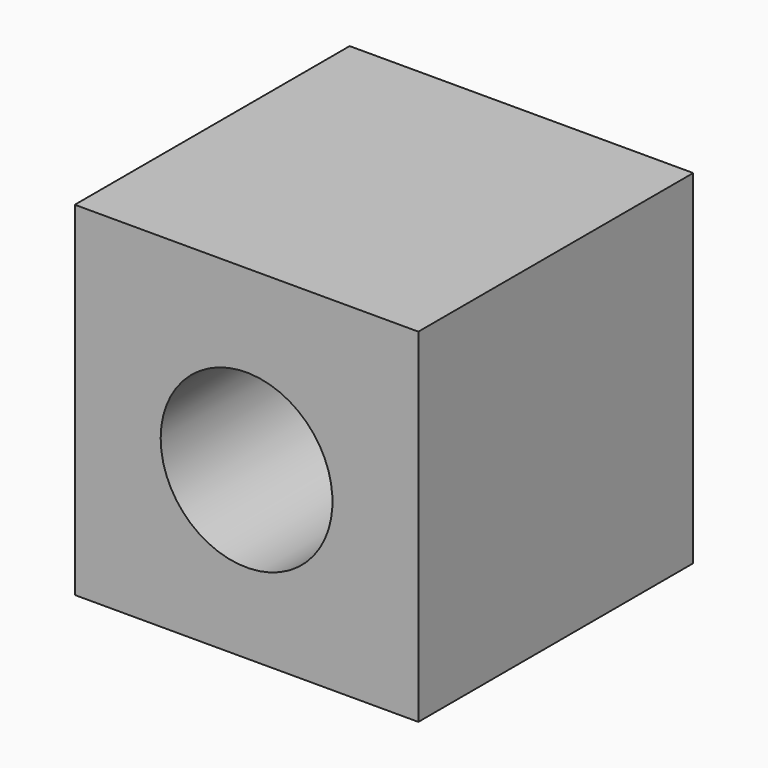
from build123d import *

# Parameters (mm, degrees)
F0_W     = 40
F0_H     = 40
F1_DEPTH = 40
F3_D     = 20


# Not quite as in the source:
# - a feature names something its author has since deleted; it is built from what else it names


with BuildPart() as f1:
    # F0 (on Front) → F1 (new body)
    with BuildSketch(Plane.XZ):
        with Locations((2.679047659, 0.6785862893)):
            Rectangle(F0_W, F0_H)
    extrude(amount=F1_DEPTH)

    # F3 (through all)
    with Locations(Plane.XZ.offset(40)):
        with Locations((2.679047659, 0)):
            Hole(F3_D / 2)


solid = f1.part
